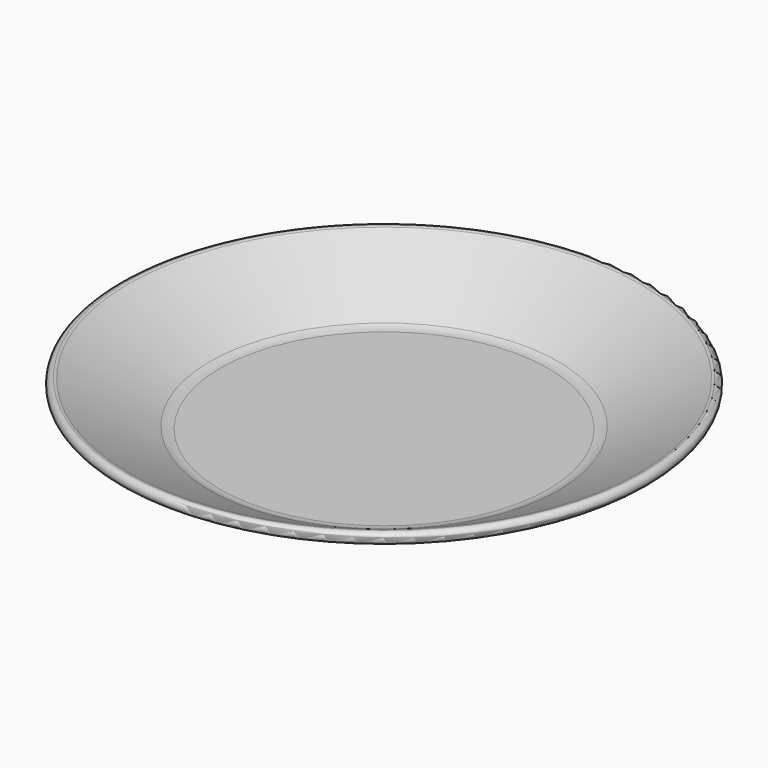
from build123d import *

# Parameters (mm, degrees)
F0_R     = 38.8061370384
F2_R     = 63.433920718
F4_T     = -2.54
F5_R     = 1.26999
F6_R     = 31.6978703438
F7_DEPTH = 1.27
F9_R     = 5.08


# Not quite as in the source:
# - a fillet or chamfer that OpenCascade refuses, or shapes differently, is made with other operations: its cross-section is extruded or revolved along the edge and cut away or added
# - a fillet or chamfer is up to 0.001 mm smaller than in the source, because OpenCascade refuses the exact size


with BuildPart() as f3:
    # F0 (on Top) → F3 section 0
    with BuildSketch(Plane.XY):
        Circle(F0_R)
    # F2 (on offset) → F3 section 1
    with BuildSketch(Plane.XY.offset(12.7)):
        Circle(F2_R)
    loft()

    # F4
    f4_openings = [f3.faces().sort_by_distance(p)[0] for p in [
        (0, 0, 12.7),
    ]]
    offset(amount=F4_T, openings=f4_openings, kind=Kind.INTERSECTION)

    # F5 (radius 1.27 in the source; OpenCascade refuses exactly that, so slightly less here)
    f5_edges = [f3.edges().sort_by_distance(p)[0] for p in [
        (-63.433921, 0, 12.7),
        (-57.892016, 0, 12.7),
    ]]
    fillet(f5_edges, radius=F5_R)

    # F6 (on face) → F7 (cut)
    with BuildSketch(Plane(origin=(0, 0, 0), x_dir=(1, 0, 0), z_dir=(0, 0, -1))):
        Circle(F6_R)
    extrude(amount=-F7_DEPTH, mode=Mode.SUBTRACT)

    # F8: fillet of radius 5.08 on 2 edges, made by hand

    # F8_s1 → F8_t2 (revolve, cut)
    with BuildSketch(Plane.XZ):
        with BuildLine():
            ThreePointArc((35.0579745088, 0), (33.2619232846, 0.3280951188), (31.6978703438, 1.27))
            Line((31.6978703438, 1.27), (31.6978703438, 0))
            Line((31.6978703438, 0), (35.0579745088, 0))
        make_face()
    revolve(axis=Axis((0, 0, 0), (0, 0, -1)), mode=Mode.SUBTRACT)

    # F8_s3 → F8_t4 (revolve, cut)
    with BuildSketch(Plane.XZ):
        with BuildLine():
            ThreePointArc((39.9017377768, 0.5649769203), (38.7713729734, 0.1432643759), (37.5734408477, 0))
            Line((37.5734408477, 0), (38.8061370384, 0))
            Line((38.8061370384, 0), (39.9017377768, 0.5649769203))
        make_face()
    revolve(axis=Axis((0, 0, 0), (0, 0, 1)), mode=Mode.SUBTRACT)

    # F9
    f9_edges = [f3.edges().sort_by_distance(p)[0] for p in [
        (-38.189789, 0, 2.54),
    ]]
    fillet(f9_edges, radius=F9_R)


solid = f3.part
